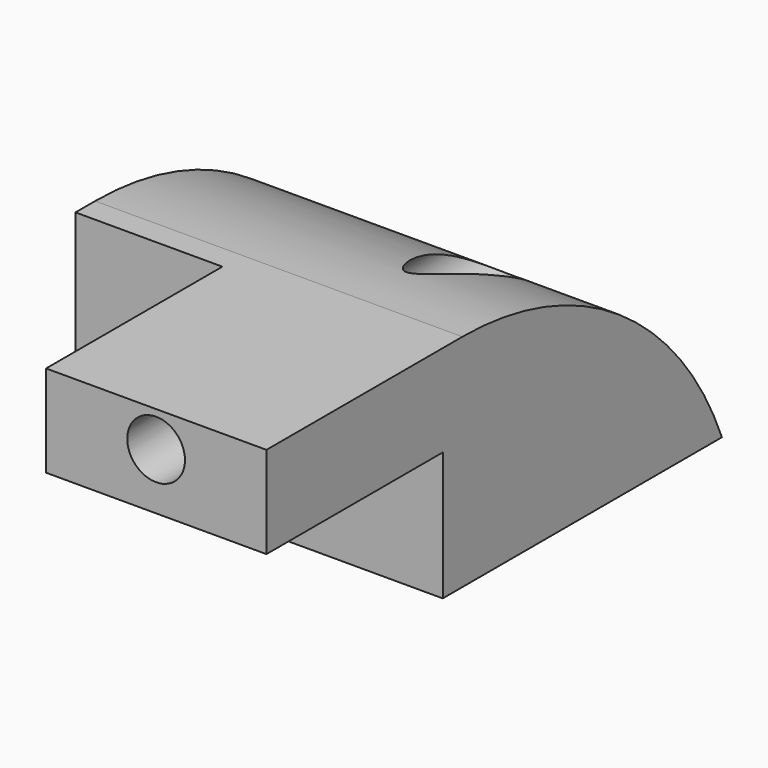
from build123d import *

# Parameters (mm, degrees)
F0_W        = 127
F0_H        = 120.65
F1_DEPTH    = 76.2
F2_T1_DEPTH = 687.8168150118
F3_W        = 76.2
F3_H        = 31.75
F4_DEPTH    = 76.2
F5_R        = 9.9779768357
F6_DEPTH    = 215.9


# Not quite as in the source:
# - a fillet or chamfer that OpenCascade refuses, or shapes differently, is made with other operations: its cross-section is extruded or revolved along the edge and cut away or added


with BuildPart() as f1:
    # F0 (on Top) → F1 (new body)
    with BuildSketch(Plane.XY):
        with Locations((25.4407467544, -4.8593845844)):
            Rectangle(F0_W, F0_H)
    extrude(amount=F1_DEPTH)

    # F2: fillet of radius 120.65 on 1 edges, made by hand

    # F2_s2 → F2_t1 (cut)
    with BuildSketch(Plane.YZ.offset(-318.4676607515)):
        with BuildLine():
            ThreePointArc((55.4656154156, 0), (11.1016993136, 55.3480836489), (-56.6977475868, 76.2))
            Line((-56.6977475868, 76.2), (55.4656154156, 76.2))
            Line((55.4656154156, 76.2), (55.4656154156, 0))
        make_face()
    extrude(amount=F2_T1_DEPTH, mode=Mode.SUBTRACT)

    # F3 (on face) → F4 (join)
    with BuildSketch(Plane.XZ.offset(65.1843845844)):
        with Locations((50.8407467544, 60.325)):
            Rectangle(F3_W, F3_H)
    extrude(amount=F4_DEPTH)

    # F5 (on face) → F6 (cut)
    with BuildSketch(Plane.XZ.offset(141.3843845844)):
        with Locations((50.7810004056, 63.9038160443)):
            Circle(F5_R)
    extrude(amount=-F6_DEPTH, mode=Mode.SUBTRACT)


solid = f1.part
